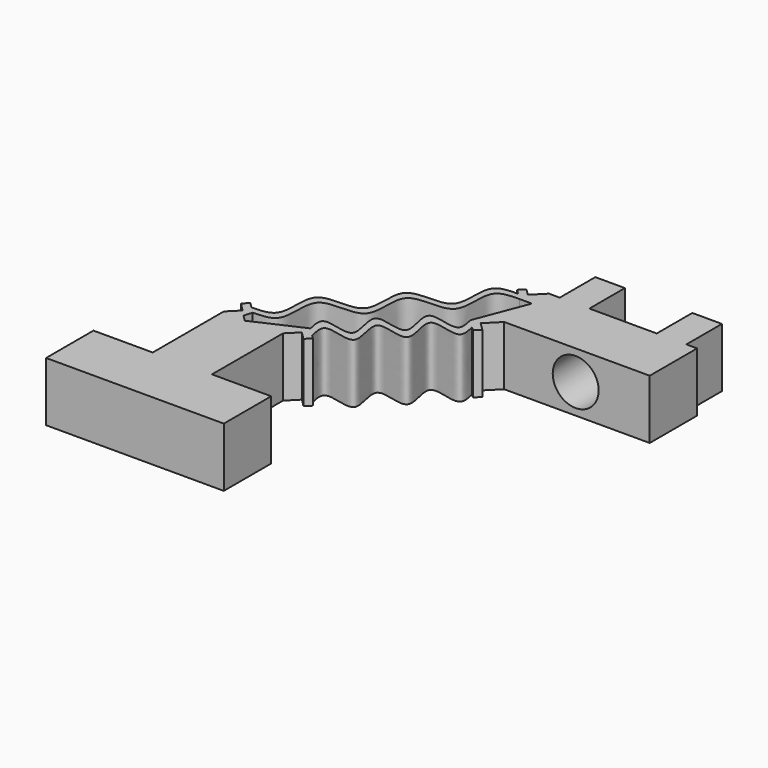
from build123d import *

# Parameters (mm, degrees)
F1_DEPTH = 4
F2_W     = 2
F2_H     = 4
F3_DEPTH = 3
F4_R     = 1.55
F5_DEPTH = 4
F8_DEPTH = 4


# Not quite as in the source:
# - ends of sketch curves that miss each other by under 0.0002 mm in the source are joined
# - the dataset's text gives a spline's control points without its knots; the knots are read off the source's solid


with BuildPart() as f1:
    # F0 (on Top) → F1 (new body)
    with BuildSketch(Plane.XY):
        with BuildLine():
            Line((4, 0), (8, 0))
            Line((8, 0), (12, 0))
            Line((12, 0), (12, 4))
            Line((12, 4), (8, 4))
            Line((8, 4), (8, 10))
            Line((8, 10), (8.7071067812, 10.7071067812))
            Line((8.7071067812, 10.7071067812), (8.1767766953, 11.2374368671))
            Line((8.1767766953, 11.2374368671), (8.5303300859, 11.5909902577))
            Line((8.5303300859, 11.5909902577), (8.7778174593, 11.3435028843))
            add(Edge.make_bspline(
                [(8.7778174593, 11.3435028843), (8.6793135956, 11.7753291065), (8.4823058683, 12.638981551), (9.7777845344, 12.3434699588), (10.6414369797, 12.1464622341), (10.8080981583, 12.3131234115)],
                knots=[0, 0, 0, 0, 0.0833326877, 0.1666653755, 0.2499980632, 0.2499980632, 0.2499980632, 0.2499980632], degree=3))
            add(Edge.make_bspline(
                [(10.8080981583, 12.3131234115), (10.9747593369, 12.4797845889), (10.7777516061, 13.3434370232), (10.4822400343, 14.6389157463), (11.7777186285, 14.343403944), (13.0731975651, 14.047893141), (12.7776849661, 15.3433688663), (12.4821771366, 16.6388585097), (13.7776618368, 16.3433013729), (15.073233045, 16.047933522), (14.8762893212, 16.9116464302), (14.7778174593, 17.3435028843)],
                knots=[0.2499980632, 0.2499980632, 0.2499980632, 0.2499980632, 0.333330751, 0.4166634387, 0.4999961264, 0.5833288142, 0.6666615019, 0.7499941897, 0.8333268774, 0.9166634387, 1, 1, 1, 1], degree=3))
            Line((14.7778174593, 17.3435028843), (14.5303300859, 17.5909902577))
            Line((14.5303300859, 17.5909902577), (14.8838834765, 17.9445436483))
            Line((14.8838834765, 17.9445436483), (15.4142135624, 17.4142135624))
            Line((15.4142135624, 17.4142135624), (16.2980970389, 18.2980970389))
            Line((16.2980970389, 18.2980970389), (26.1212241882, 18.2980970389))
            Line((26.1212241882, 18.2980970389), (26.1212241882, 22.2980970389))
            Line((26.1212241882, 22.2980970389), (16.1212241882, 22.2980970389))
            Line((16.1212241882, 22.2980970389), (15.3256809034, 21.5025539105))
            Line((15.3256809034, 21.5025539105), (15.7675746595, 21.0606601544))
            Line((15.7675746595, 21.0606601544), (15.4140212689, 20.7071067638))
            Line((15.4140212689, 20.7071067638), (15.3257290593, 20.7953989734))
            Line((15.3257290593, 20.7953989734), (15.2726959638, 20.8484320689))
            add(Edge.make_bspline(
                [(5.2727919408, 10.8485280459), (5.8157320976, 10.8611381168), (6.9016124112, 10.8863582587), (6.939442624, 12.5151787291), (6.9772728368, 14.1439991996), (8.6060933073, 14.1818294124), (10.2349137777, 14.2196596252), (10.2727439905, 15.8484800956), (10.3105742033, 17.4773005661), (11.9393946738, 17.5151307789), (13.5682151443, 17.5529609917), (13.6060453571, 19.1817814621), (13.6438755698, 20.8106019326), (14.7297558835, 20.8358220745), (15.2726959638, 20.8484320689)],
                knots=[0, 0, 0, 0, 0.0833333333, 0.1666666667, 0.25, 0.3333333333, 0.4166666667, 0.5, 0.5833333333, 0.6666666667, 0.75, 0.8333333333, 0.9166666667, 1, 1, 1, 1], degree=3))
            Line((5.2727919408, 10.8485280459), (5.6282136765, 10.4931061393))
            Line((5.6282136765, 10.4931061393), (5.2746603207, 10.1395527139))
            Line((5.2746603207, 10.1395527139), (4.7071065842, 10.7071067232))
            Line((4.7071065842, 10.7071067232), (4, 10))
            Line((4, 10), (4, 4))
            Line((4, 4), (0, 4))
            Line((0, 4), (0, 0))
            Line((0, 0), (4, 0))
        make_face()
        Polygon((8.1767766953, 11.2374368671), (8.7071067812, 10.7071067812), (9.2374368671, 10.1767766953), (9.5909902577, 10.5303300859), (9.3435028843, 10.7778174593), (9.0606601718, 11.0606601718), (8.7778174593, 11.3435028843), (8.5303300859, 11.5909902577), align=None)
        Polygon((4.1395527627, 11.2746608175), (4.7071065842, 10.7071067232), (4.8838832621, 10.8838834359), (5.0606599574, 11.0606601312), (4.848527974, 11.2727922166), (4.7954948913, 11.3258253248), (4.4931062383, 11.6282141232), align=None)
        Polygon((4.8838832621, 10.8838834359), (4.7071065842, 10.7071067232), (5.2746603207, 10.1395527139), (5.6282136765, 10.4931061393), (5.2727919408, 10.8485280459), (5.0606599574, 11.0606601312), align=None)
        with BuildLine():
            Line((4.848527974, 11.2727922166), (5.0606599574, 11.0606601312))
            Line((5.0606599574, 11.0606601312), (5.2727919408, 10.8485280459))
            add(Edge.make_bspline(
                [(5.2727919408, 10.8485280459), (5.8157320976, 10.8611381168), (6.9016124112, 10.8863582587), (6.939442624, 12.5151787291), (6.9772728368, 14.1439991996), (8.6060933073, 14.1818294124), (10.2349137777, 14.2196596252), (10.2727439905, 15.8484800956), (10.3105742033, 17.4773005661), (11.9393946738, 17.5151307789), (13.5682151443, 17.5529609917), (13.6060453571, 19.1817814621), (13.6438755698, 20.8106019326), (14.7297558835, 20.8358220745), (15.2726960403, 20.8484321454)],
                knots=[0, 0, 0, 0, 0.0833333333, 0.1666666667, 0.25, 0.3333333333, 0.4166666667, 0.5, 0.5833333333, 0.6666666667, 0.75, 0.8333333333, 0.9166666667, 1, 1, 1, 1], degree=3))
            Line((15.2726960403, 20.8484321454), (14.8484318951, 21.2726961376))
            add(Edge.make_bspline(
                [(4.848527974, 11.2727922166), (5.3914681818, 11.2854023385), (6.4773484955, 11.3106224803), (6.5151787083, 12.9394429508), (6.5530089211, 14.5682634213), (8.1818293915, 14.6060936341), (9.810649862, 14.6439238468), (9.8484800748, 16.2727443173), (9.8863102876, 17.9015647878), (11.5151307581, 17.9393950006), (13.1439512285, 17.9772252134), (13.1817814413, 19.6060456838), (13.2196116541, 21.2348661543), (14.3054919677, 21.2600862962), (14.8484318951, 21.2726961376)],
                knots=[0, 0, 0, 0, 0.0833333333, 0.1666666667, 0.25, 0.3333333333, 0.4166666667, 0.5, 0.5833333333, 0.6666666667, 0.75, 0.8333333333, 0.9166666667, 1, 1, 1, 1], degree=3))
        make_face()
        with BuildLine():
            add(Edge.make_bspline(
                [(8.7778174593, 11.3435028843), (8.6793135956, 11.7753291065), (8.4823058683, 12.638981551), (9.7777845344, 12.3434699588), (10.6414369797, 12.1464622341), (10.8080981583, 12.3131234115)],
                knots=[0, 0, 0, 0, 0.0833326877, 0.1666653755, 0.2499980632, 0.2499980632, 0.2499980632, 0.2499980632], degree=3))
            Line((8.7778174593, 11.3435028843), (9.0606601718, 11.0606601718))
            Line((9.0606601718, 11.0606601718), (9.3435028843, 10.7778174593))
            add(Edge.make_bspline(
                [(9.3435028843, 10.7778174593), (9.2449990206, 11.2096436816), (9.0479912932, 12.0732961261), (10.3434699594, 11.7777845339), (11.6389486273, 11.4822729468), (11.343437031, 12.7777515982), (11.0479254593, 14.0732303213), (12.3434040535, 13.777718519), (13.6388829901, 13.482207716), (13.343370391, 14.7776834413), (13.0478625616, 16.0731730848), (14.3433472618, 15.7776159479), (15.6389184699, 15.4822480971), (15.4419747461, 16.3459610052), (15.3435028843, 16.7778174593)],
                knots=[0, 0, 0, 0, 0.0833326877, 0.1666653755, 0.2499980632, 0.333330751, 0.4166634387, 0.4999961264, 0.5833288142, 0.6666615019, 0.7499941897, 0.8333268774, 0.9166634387, 1, 1, 1, 1], degree=3))
            Line((15.3435028843, 16.7778174593), (14.7778174593, 17.3435028843))
            add(Edge.make_bspline(
                [(10.8080981583, 12.3131234115), (10.9747593369, 12.4797845889), (10.7777516061, 13.3434370232), (10.4822400343, 14.6389157463), (11.7777186285, 14.343403944), (13.0731975651, 14.047893141), (12.7776849661, 15.3433688663), (12.4821771366, 16.6388585097), (13.7776618368, 16.3433013729), (15.073233045, 16.047933522), (14.8762893212, 16.9116464302), (14.7778174593, 17.3435028843)],
                knots=[0.2499980632, 0.2499980632, 0.2499980632, 0.2499980632, 0.333330751, 0.4166634387, 0.4999961264, 0.5833288142, 0.6666615019, 0.7499941897, 0.8333268774, 0.9166634387, 1, 1, 1, 1], degree=3))
        make_face()
        Polygon((14.7778174593, 17.3435028843), (15.3435028843, 16.7778174593), (15.5909902577, 16.5303300859), (15.9445436483, 16.8838834765), (15.4142135624, 17.4142135624), (14.8838834765, 17.9445436483), (14.5303300859, 17.5909902577), align=None)
        Polygon((14.7953989734, 21.3257290593), (14.8484318951, 21.2726961376), (15.2726959638, 20.8484320689), (15.3257290593, 20.7953989734), (15.4140212689, 20.7071067638), (15.7675746595, 21.0606601544), (15.3256809034, 21.5025539105), (14.8837871473, 21.9444476667), (14.5302337567, 21.5908942761), align=None)
    extrude(amount=F1_DEPTH)

    # F2 (on face) → F3 (join)
    with BuildSketch(Plane(origin=(0, 22.2980970389, 0), x_dir=(-1, 0, 0), z_dir=(0, 1, 0))):
        with Locations((-24.3962241882, 2)):
            Rectangle(F2_W, F2_H)
        with Locations((-17.8462241882, 2)):
            Rectangle(F2_W, F2_H)
    extrude(amount=F3_DEPTH)

    # F4 (on face) → F5 (cut)
    with BuildSketch(Plane(origin=(0, 22.2980970389, 0), x_dir=(-1, 0, 0), z_dir=(0, 1, 0))):
        with Locations((-21.1212241882, 2)):
            Circle(F4_R)
    extrude(amount=-F5_DEPTH, mode=Mode.SUBTRACT)


with BuildPart() as f6_1:
    # F6: copy of F1
    add(f1.part)


with BuildPart() as f8_tool:
    # F7 (on face) → F8 (new body)
    with BuildSketch(Plane.XY.offset(4)):
        with BuildLine():
            add(Edge.make_bspline(
                [(5.2727919408, 10.8485280459), (5.8157320976, 10.8611381168), (6.9016124112, 10.8863582587), (6.939442624, 12.5151787291), (6.9772728368, 14.1439991996), (8.6060933073, 14.1818294124), (10.2349137777, 14.2196596252), (10.2727439905, 15.8484800956), (10.3105742033, 17.4773005661), (11.9393946738, 17.5151307789), (13.5682151443, 17.5529609917), (13.6060453571, 19.1817814621), (13.6438755698, 20.8106019326), (14.7297558835, 20.8358220745), (15.2726960403, 20.8484321454)],
                knots=[0, 0, 0, 0, 0.0833333333, 0.1666666667, 0.25, 0.3333333333, 0.4166666667, 0.5, 0.5833333333, 0.6666666667, 0.75, 0.8333333333, 0.9166666667, 1, 1, 1, 1], degree=3))
            Line((5.2727919408, 10.8485280459), (5.1121239237, 10.2786554684))
            Line((5.1121239237, 10.2786554684), (5.5245361812, 9.866243292))
            Line((5.5245361812, 9.866243292), (8.7778174593, 11.3435028843))
            add(Edge.make_bspline(
                [(8.7778174593, 11.3435028843), (8.6793135956, 11.7753291065), (8.4823058683, 12.638981551), (9.7777845344, 12.3434699588), (11.0732632024, 12.0479583718), (10.7777516061, 13.3434370232), (10.4822400343, 14.6389157463), (11.7777186285, 14.343403944), (13.0731975651, 14.047893141), (12.7776849661, 15.3433688663), (12.4821771366, 16.6388585097), (13.7776618368, 16.3433013729), (15.073233045, 16.047933522), (14.8762893212, 16.9116464302), (14.7778174593, 17.3435028843)],
                knots=[0, 0, 0, 0, 0.0833326877, 0.1666653755, 0.2499980632, 0.333330751, 0.4166634387, 0.4999961264, 0.5833288142, 0.6666615019, 0.7499941897, 0.8333268774, 0.9166634387, 1, 1, 1, 1], degree=3))
            Line((14.7778174593, 17.3435028843), (16.1212241882, 20.8484321454))
            Line((16.1212241882, 20.8484321454), (15.2726960403, 20.8484321454))
        make_face()
    extrude(amount=-F8_DEPTH)


with BuildPart() as f1_1:
    add(f1.part)

    # F8: cut by f8_tool
    add(f8_tool.part, mode=Mode.SUBTRACT)


with BuildPart() as f6_1_1:
    add(f6_1.part)

    # F8: cut by f8_tool
    add(f8_tool.part, mode=Mode.SUBTRACT)


solid = Compound([f1_1.part, f6_1_1.part])
